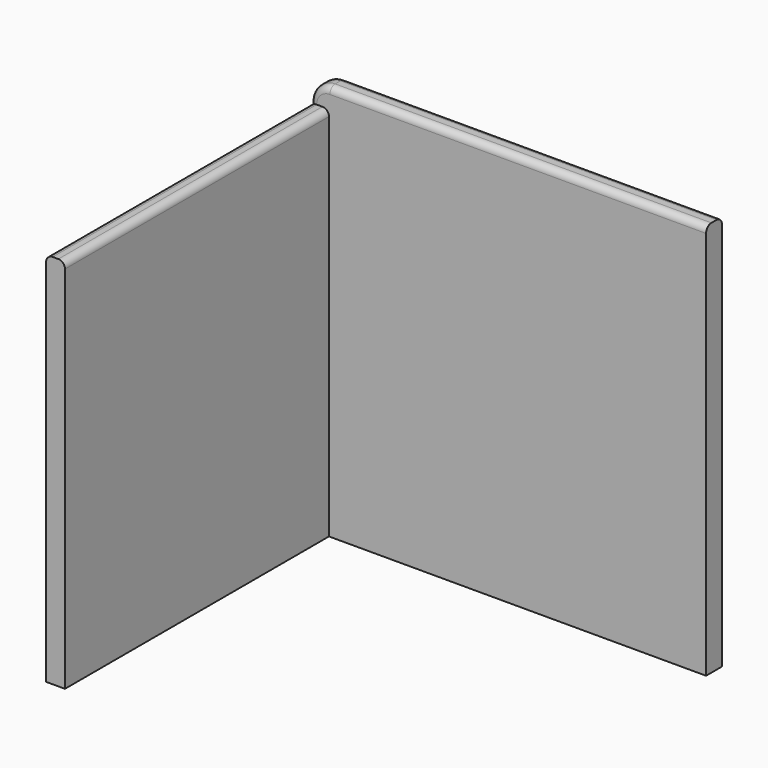
from build123d import *

# Parameters (mm, degrees)
F0_W     = 120
F0_H     = 120
F1_DEPTH = 6
F2_R     = 6
F3_W     = 5.722270757
F3_H     = 114
F4_DEPTH = 100
F5_R     = 2
F6_R     = 1.99999


# Not quite as in the source:
# - a fillet or chamfer is up to 0.001 mm smaller than in the source, because OpenCascade refuses the exact size


with BuildPart() as f1:
    # F0 (on Front) → F1 (new body)
    with BuildSketch(Plane.XZ):
        with Locations((3.6820918322, -11.3266304067)):
            Rectangle(F0_W, F0_H)
    extrude(amount=F1_DEPTH)

    # F2
    f2_edges = [f1.edges().sort_by_distance(p)[0] for p in [
        (-56.317908, -3, 48.67337),
    ]]
    fillet(f2_edges, radius=F2_R)

    # F3 (on face) → F4 (join)
    with BuildSketch(Plane.XZ.offset(6)):
        with Locations((-53.4567727894, -14.3266304067)):
            Rectangle(F3_W, F3_H)
    extrude(amount=F4_DEPTH)

    # F5
    f5_edges = [f1.edges().sort_by_distance(p)[0] for p in [
        (-56.317908, -56, 42.67337),
        (-50.595637, -56, 42.67337),
    ]]
    fillet(f5_edges, radius=F5_R)

    # F6 (radius 2 in the source; OpenCascade refuses exactly that, so slightly less here)
    f6_edges = [f1.edges().sort_by_distance(p)[0] for p in [
        (6.682092, -6, 48.67337),
        (6.682092, 0, 48.67337),
    ]]
    fillet(f6_edges, radius=F6_R)


solid = f1.part
